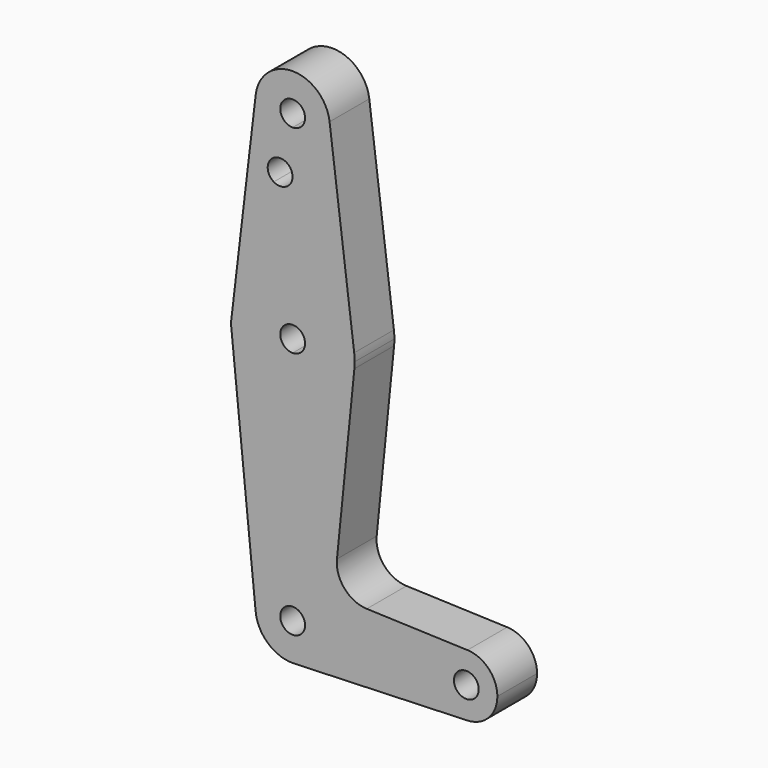
from build123d import *

# Parameters (mm, degrees)
F1_DEPTH = 12.7


with BuildPart() as f1:
    # F0 (on Front) → F1 (new body)
    with BuildSketch(Plane.XZ):
        with BuildLine():
            Line((0, 79.375), (0, 89.5573869348))
            Line((0, 89.5573869348), (0, 100.0252))
            Line((0, 100.0252), (-0.0357827719, 100.0252))
            ThreePointArc((-0.0357827719, 100.0252), (-1.6439653205, 97.2637315367), (-4.8393784091, 97.2997089891))
            Line((-4.8393784091, 97.2997089891), (-4.8393784091, 78.6193928983))
            ThreePointArc((-4.8393784091, 78.6193928983), (-2.4490062004, 79.1849607469), (0, 79.375))
        make_face()
        with BuildLine():
            Line((0, 100.0252), (0, 89.5573869348))
            Line((0, 89.5573869348), (0, 79.375))
            ThreePointArc((0, 79.375), (10.5003255158, 75.40625), (15.7504882737, 65.484375))
            Line((15.7504882737, 65.484375), (9.4502929642, 115.490625))
            ThreePointArc((9.4502929642, 115.490625), (9.5063048942, 114.896483242), (9.525, 114.3))
            ThreePointArc((9.525, 114.3), (6.7351920908, 107.5648079092), (0, 104.775))
            Line((0, 104.775), (0, 100.0252))
        make_face()
        with BuildLine():
            Line((-0.0357827719, 100.0252), (0, 100.0252))
            Line((0, 100.0252), (0, 104.775))
            ThreePointArc((0, 104.775), (-7.1202192788, 107.9732233782), (-9.4589053806, 115.4201490977))
            Line((-9.4589053806, 115.4201490977), (-14.9877324754, 68.7329246359))
            ThreePointArc((-14.9877324754, 68.7329246359), (-11.0776416797, 74.8710808553), (-4.8393784091, 78.6193928983))
            Line((-4.8393784091, 78.6193928983), (-4.8393784091, 97.2997089891))
            ThreePointArc((-4.8393784091, 97.2997089891), (-4.7776002233, 102.7866684633), (-0.0357827719, 100.0252))
        make_face()
        with BuildLine():
            ThreePointArc((15.7504882737, 65.484375), (10.5003255158, 75.40625), (0, 79.375))
            Line((0, 79.375), (0, 66.675))
            ThreePointArc((0, 66.675), (2.2450640303, 65.7450640303), (3.175, 63.5))
            ThreePointArc((3.175, 63.5), (2.2450640303, 61.2549359697), (0, 60.325))
            Line((0, 60.325), (0, 47.625))
            ThreePointArc((0, 47.625), (10.6492737428, 51.7267849017), (15.7954255641, 61.9125))
            ThreePointArc((15.7954255641, 61.9125), (15.8550939106, 62.7052534459), (15.875, 63.5))
            ThreePointArc((15.875, 63.5), (15.8438414904, 64.4941387366), (15.7504882737, 65.484375))
        make_face()
        with BuildLine():
            Line((0, 66.675), (0, 79.375))
            ThreePointArc((0, 79.375), (-2.4490062004, 79.1849607469), (-4.8393784091, 78.6193928983))
            ThreePointArc((-4.8393784091, 78.6193928983), (-11.0776416797, 74.8710808553), (-14.9877324754, 68.7329246359))
            Line((-14.9877324754, 68.7329246359), (-15.7954255641, 61.9125))
            ThreePointArc((-15.7954255641, 61.9125), (-10.6492737428, 51.7267849017), (0, 47.625))
            Line((0, 47.625), (0, 60.325))
            ThreePointArc((0, 60.325), (-3.175, 63.5), (0, 66.675))
        make_face()
        with BuildLine():
            ThreePointArc((-9.4589053806, 115.4201490977), (-7.1202192788, 107.9732233782), (0, 104.775))
            ThreePointArc((0, 104.775), (6.7351920908, 107.5648079092), (9.525, 114.3))
            ThreePointArc((9.525, 114.3), (9.5063048942, 114.896483242), (9.4502929642, 115.490625))
            ThreePointArc((9.4502929642, 115.490625), (-0.0355000934, 123.8249338446), (-9.4589053806, 115.4201490977))
        make_face()
        with BuildLine():
            ThreePointArc((3.175, 114.3), (2.2450640303, 112.0549359697), (0, 111.125))
            ThreePointArc((0, 111.125), (-2.2450640303, 116.5450640303), (3.175, 114.3))
        make_face(mode=Mode.SUBTRACT)
        with BuildLine():
            ThreePointArc((15.7954255641, 61.9125), (10.6492737428, 51.7267849017), (0, 47.625))
            Line((0, 47.625), (0, 9.525))
            ThreePointArc((0, 9.525), (6.7351920908, 6.7351920908), (9.525, 0))
            Line((9.525, 0), (36.5125, 0))
            ThreePointArc((36.5125, 0), (38.9384772185, 5.7120069047), (44.7334821429, 7.9324362036))
            Line((44.7334821429, 7.9324362036), (18.9676000005, 8.8532337108))
            ThreePointArc((18.9676000005, 8.8532337108), (13.2611998974, 11.5713591498), (11.3411865923, 17.5933818124))
            Line((11.3411865923, 17.5933818124), (15.7954255641, 61.9125))
        make_face()
        with BuildLine():
            Line((0, 9.525), (0, 47.625))
            ThreePointArc((0, 47.625), (-10.6492737428, 51.7267849017), (-15.7954255641, 61.9125))
            Line((-15.7954255641, 61.9125), (-9.4772553384, -0.9525))
            ThreePointArc((-9.4772553384, -0.9525), (-7.063929059, 6.3895642457), (0, 9.525))
        make_face()
        with BuildLine():
            ThreePointArc((9.525, 0), (6.7351920908, 6.7351920908), (0, 9.525))
            Line((0, 9.525), (0, 3.175))
            ThreePointArc((0, 3.175), (2.2450640303, 2.2450640303), (3.175, 0))
            Line((3.175, 0), (9.525, 0))
        make_face()
        with BuildLine():
            Line((0, 3.175), (0, 9.525))
            ThreePointArc((0, 9.525), (-7.063929059, 6.3895642457), (-9.4772553384, -0.9525))
            ThreePointArc((-9.4772553384, -0.9525), (-6.2623833816, -7.1769199091), (0.3401785714, -9.5189234444))
            ThreePointArc((0.3401785714, -9.5189234444), (6.8544082857, -6.6138273378), (9.525, 0))
            Line((9.525, 0), (3.175, 0))
            ThreePointArc((3.175, 0), (-2.2450640303, -2.2450640303), (0, 3.175))
        make_face()
        with BuildLine():
            Line((36.5125, 0), (9.525, 0))
            ThreePointArc((9.525, 0), (6.8544082857, -6.6138273378), (0.3401785714, -9.5189234444))
            Line((0.3401785714, -9.5189234444), (44.7334821429, -7.9324362036))
            ThreePointArc((44.7334821429, -7.9324362036), (38.9384772185, -5.7120069047), (36.5125, 0))
        make_face()
        with BuildLine():
            ThreePointArc((44.7334821429, 7.9324362036), (38.9384772185, 5.7120069047), (36.5125, 0))
            ThreePointArc((36.5125, 0), (38.9384772185, -5.7120069047), (44.7334821429, -7.9324362036))
            ThreePointArc((44.7334821429, -7.9324362036), (50.1620069047, -5.5115227815), (52.3875, 0))
            ThreePointArc((52.3875, 0), (50.1620069047, 5.5115227815), (44.7334821429, 7.9324362036))
        make_face()
        with BuildLine():
            ThreePointArc((47.625, 0), (44.45, -3.175), (41.275, 0))
            ThreePointArc((41.275, 0), (44.45, 3.175), (47.625, 0))
        make_face(mode=Mode.SUBTRACT)
    extrude(amount=F1_DEPTH)


solid = f1.part
